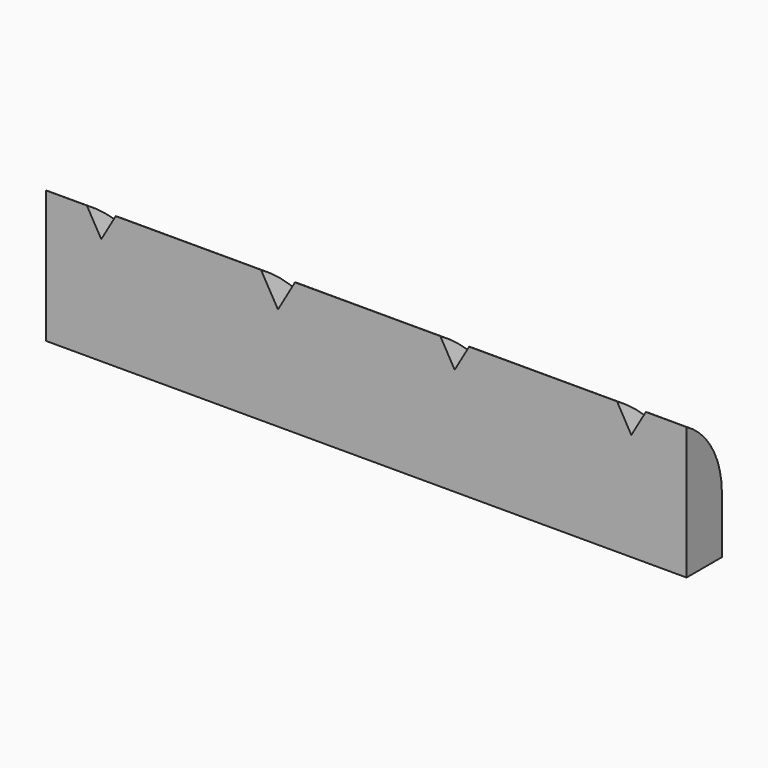
from build123d import *

# Parameters (mm, degrees)
F0_W        = 36.83
F0_H        = 2.54
F1_DEPTH    = 7.62
F3_T1_DEPTH = 58.8270452561
F4_DEPTH    = 25.4


# Not quite as in the source:
# - a fillet or chamfer that OpenCascade refuses, or shapes differently, is made with other operations: its cross-section is extruded or revolved along the edge and cut away or added


with BuildPart() as f1:
    # F0 (on Top) → F1 (new body)
    with BuildSketch(Plane.XY):
        with Locations((-0.635, 1.27)):
            Rectangle(F0_W, F0_H)
    extrude(amount=F1_DEPTH)

    # F3: fillet of radius 5.08 on 1 edges, made by hand

    # F3_s2 → F3_t1 (cut)
    with BuildSketch(Plane.YZ.offset(-30.0485226281)):
        with BuildLine():
            ThreePointArc((2.54, 3.2205909488), (1.8594090512, 5.7605909488), (0, 7.62))
            Line((0, 7.62), (2.54, 7.62))
            Line((2.54, 7.62), (2.54, 3.2205909488))
        make_face()
    extrude(amount=F3_T1_DEPTH, mode=Mode.SUBTRACT)

    # F2 (on face) → F4 (cut)
    with BuildSketch(Plane.XZ):
        Polygon((-15.875, 6.1822954744), (-15.0449409051, 7.62), (-16.7050590949, 7.62), align=None)
        Polygon((-4.7382939367, 7.62), (-6.6917060633, 7.62), (-5.715, 5.9282954744), align=None)
        Polygon((5.2750590949, 7.62), (3.6149409051, 7.62), (4.445, 6.1822954744), align=None)
        Polygon((15.4350590949, 7.62), (13.7749409051, 7.62), (14.605, 6.1822954744), align=None)
    extrude(amount=-F4_DEPTH, mode=Mode.SUBTRACT)


solid = f1.part
